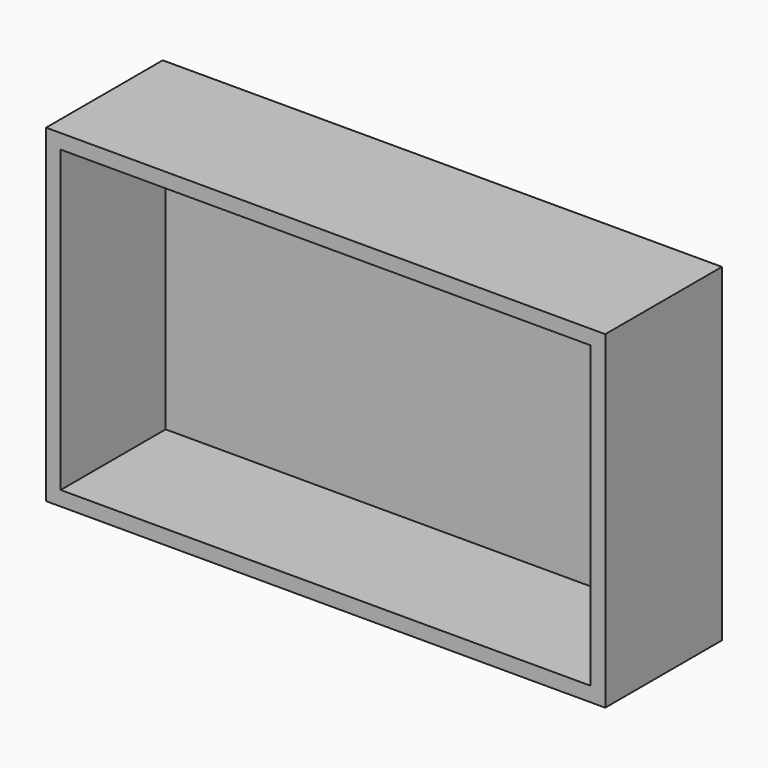
from build123d import *

# Parameters (mm, degrees)
F0_W     = 97.3927639425
F0_H     = 57.274825871
F1_DEPTH = 25.4
F2_T     = -2.54


# Not quite as in the source:
# - the program builds the solid bodies; features that only make, move or delete a surface that nothing else refers to are left out


with BuildPart() as f1:
    # F0 (on Front) → F1 (new body)
    with BuildSketch(Plane.XZ):
        with Locations((7.3790643364, -10.254021734)):
            Rectangle(F0_W, F0_H)
    extrude(amount=F1_DEPTH)

    # F2
    f2_openings = [f1.faces().sort_by_distance(p)[0] for p in [
        (7.379064, -25.4, -10.254022),
    ]]
    offset(amount=F2_T, openings=f2_openings)


solid = f1.part
